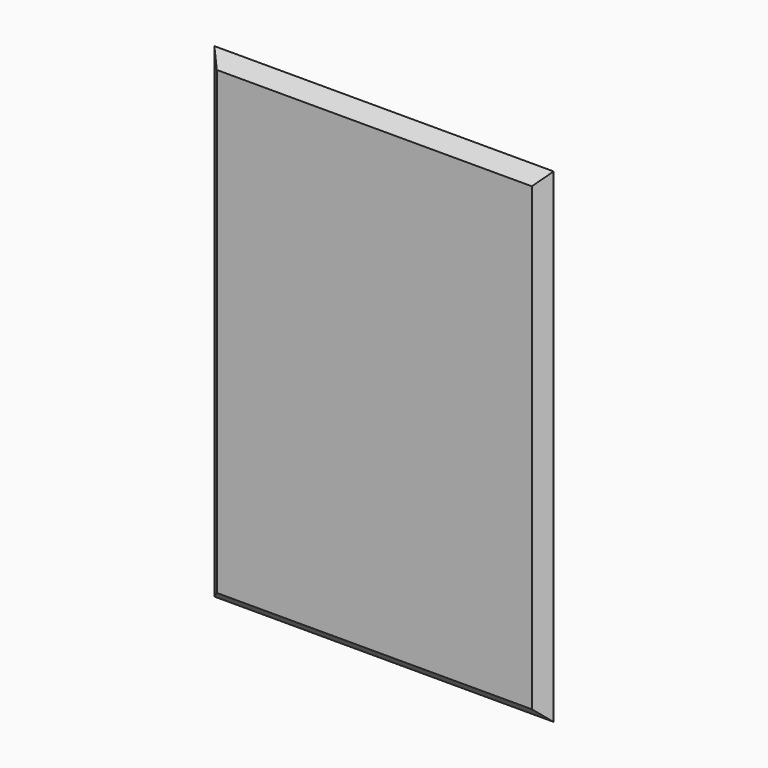
from build123d import *

# Parameters (mm, degrees)
F0_W     = 177.8
F0_H     = 254
F1_DEPTH = 6.35
F2_SIZE2 = 6.34999
F2_SIZE  = 6.34999


# Not quite as in the source:
# - a fillet or chamfer is up to 0.001 mm smaller than in the source, because OpenCascade refuses the exact size


with BuildPart() as f1:
    # F0 (on Front) → F1 (new body)
    with BuildSketch(Plane.XZ):
        with Locations((-61.3160093542, -4.4609885663)):
            Rectangle(F0_W, F0_H)
    extrude(amount=F1_DEPTH)

    # F2 (size 6.35 and 6.35 in the source; OpenCascade refuses exactly that, so slightly less here)
    f2_edges = [f1.edges().sort_by_distance(p)[0] for p in [
        (-61.316009, -6.35, 122.539011),
        (-150.216009, -6.35, -4.460989),
        (-61.316009, -6.35, -131.460989),
        (27.583991, -6.35, -4.460989),
    ]]
    chamfer(f2_edges, length=F2_SIZE, length2=F2_SIZE2)


solid = f1.part
